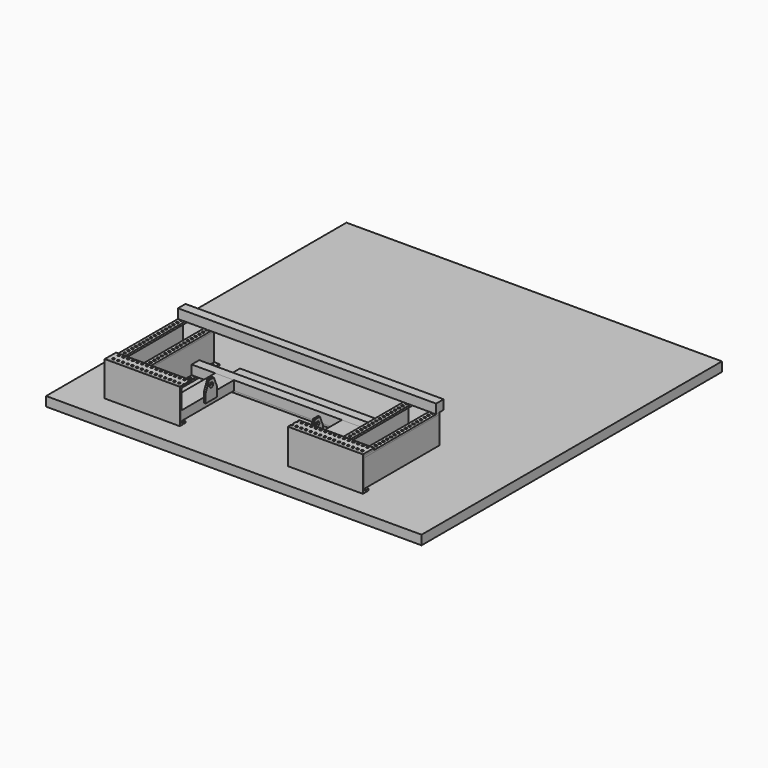
from build123d import *

# Parameters (mm, degrees)
F0_W      = 1016
F0_H      = 1016
F1_DEPTH  = 25.4
F2_W      = 698.5
F2_H      = 88.9
F3_DEPTH  = 5.08
F4_W      = 698.5
F4_H      = 38.1
F4_R      = 3.175
F5_DEPTH  = 5.08
F6_W      = 698.5
F6_H      = 19.05
F6_R      = 3.175
F7_DEPTH  = 5.08
F8_W      = 5.08
F8_H      = 73.66
F9_DEPTH  = 254
F10_W     = 19.05
F10_H     = 254
F10_R     = 3.175
F11_DEPTH = 5.08
F12_W     = 19.05
F12_H     = 254
F12_R     = 3.175
F13_DEPTH = 5.08
F15_W     = 698.5
F15_H     = 25.4
F16_DEPTH = 25.4
F17_W     = 387.35
F17_H     = 254
F18_DEPTH = 12.7
F19_W     = 292.1
F19_H     = 38.1
F20_DEPTH = 165.101
F21_W     = 292.1
F21_H     = 33.02
F22_DEPTH = 63.5
F23_W     = 50.8
F23_H     = 25.4
F24_DEPTH = 177.8
F25_W     = 520.7
F25_H     = 25.4
F26_DEPTH = 25.4
F27_W     = 38.1
F27_H     = 25.4
F27_R     = 6.35
F28_DEPTH = 5.08


with BuildPart() as f1:
    # F0 (on Top) → F1 (new body)
    with BuildSketch(Plane.XY):
        Rectangle(F0_W, F0_H)
    extrude(amount=F1_DEPTH)


with BuildPart() as f3:
    # F2 (on face) → F3 (new body)
    with BuildSketch(Plane.XZ.offset(508)):
        with Locations((0, 120.65)):
            Rectangle(F2_W, F2_H)
    extrude(amount=-F3_DEPTH)

    # F6 (on face) → F7 (join)
    with BuildSketch(Plane(origin=(0, 0, 76.2), x_dir=(1, 0, 0), z_dir=(0, 0, -1))):
        with Locations((0, 498.475)):
            Rectangle(F6_W, F6_H)
        with Locations((-336.55, 495.935)):
            Circle(F6_R, mode=Mode.SUBTRACT)
        with Locations((-323.85, 495.935)):
            Circle(F6_R, mode=Mode.SUBTRACT)
        with Locations((-311.15, 495.935)):
            Circle(F6_R, mode=Mode.SUBTRACT)
        with Locations((-298.45, 495.935)):
            Circle(F6_R, mode=Mode.SUBTRACT)
        with Locations((-285.75, 495.935)):
            Circle(F6_R, mode=Mode.SUBTRACT)
        with Locations((-273.05, 495.935)):
            Circle(F6_R, mode=Mode.SUBTRACT)
        with Locations((-260.35, 495.935)):
            Circle(F6_R, mode=Mode.SUBTRACT)
        with Locations((-247.65, 495.935)):
            Circle(F6_R, mode=Mode.SUBTRACT)
        with Locations((-234.95, 495.935)):
            Circle(F6_R, mode=Mode.SUBTRACT)
        with Locations((-222.25, 495.935)):
            Circle(F6_R, mode=Mode.SUBTRACT)
        with Locations((-209.55, 495.935)):
            Circle(F6_R, mode=Mode.SUBTRACT)
        with Locations((-196.85, 495.935)):
            Circle(F6_R, mode=Mode.SUBTRACT)
        with Locations((-184.15, 495.935)):
            Circle(F6_R, mode=Mode.SUBTRACT)
        with Locations((-171.45, 495.935)):
            Circle(F6_R, mode=Mode.SUBTRACT)
        with Locations((-158.75, 495.935)):
            Circle(F6_R, mode=Mode.SUBTRACT)
        with Locations((-146.05, 495.935)):
            Circle(F6_R, mode=Mode.SUBTRACT)
        with Locations((-133.35, 495.935)):
            Circle(F6_R, mode=Mode.SUBTRACT)
        with Locations((-120.65, 495.935)):
            Circle(F6_R, mode=Mode.SUBTRACT)
        with Locations((-107.95, 495.935)):
            Circle(F6_R, mode=Mode.SUBTRACT)
        with Locations((-95.25, 495.935)):
            Circle(F6_R, mode=Mode.SUBTRACT)
        with Locations((-82.55, 495.935)):
            Circle(F6_R, mode=Mode.SUBTRACT)
        with Locations((-69.85, 495.935)):
            Circle(F6_R, mode=Mode.SUBTRACT)
        with Locations((-57.15, 495.935)):
            Circle(F6_R, mode=Mode.SUBTRACT)
        with Locations((-44.45, 495.935)):
            Circle(F6_R, mode=Mode.SUBTRACT)
        with Locations((-31.75, 495.935)):
            Circle(F6_R, mode=Mode.SUBTRACT)
        with Locations((-19.05, 495.935)):
            Circle(F6_R, mode=Mode.SUBTRACT)
        with Locations((-6.35, 495.935)):
            Circle(F6_R, mode=Mode.SUBTRACT)
        with Locations((6.35, 495.935)):
            Circle(F6_R, mode=Mode.SUBTRACT)
        with Locations((19.05, 495.935)):
            Circle(F6_R, mode=Mode.SUBTRACT)
        with Locations((31.75, 495.935)):
            Circle(F6_R, mode=Mode.SUBTRACT)
        with Locations((44.45, 495.935)):
            Circle(F6_R, mode=Mode.SUBTRACT)
        with Locations((57.15, 495.935)):
            Circle(F6_R, mode=Mode.SUBTRACT)
        with Locations((69.85, 495.935)):
            Circle(F6_R, mode=Mode.SUBTRACT)
        with Locations((82.55, 495.935)):
            Circle(F6_R, mode=Mode.SUBTRACT)
        with Locations((95.25, 495.935)):
            Circle(F6_R, mode=Mode.SUBTRACT)
        with Locations((107.95, 495.935)):
            Circle(F6_R, mode=Mode.SUBTRACT)
        with Locations((120.65, 495.935)):
            Circle(F6_R, mode=Mode.SUBTRACT)
        with Locations((133.35, 495.935)):
            Circle(F6_R, mode=Mode.SUBTRACT)
        with Locations((146.05, 495.935)):
            Circle(F6_R, mode=Mode.SUBTRACT)
        with Locations((158.75, 495.935)):
            Circle(F6_R, mode=Mode.SUBTRACT)
        with Locations((171.45, 495.935)):
            Circle(F6_R, mode=Mode.SUBTRACT)
        with Locations((184.15, 495.935)):
            Circle(F6_R, mode=Mode.SUBTRACT)
        with Locations((196.85, 495.935)):
            Circle(F6_R, mode=Mode.SUBTRACT)
        with Locations((209.55, 495.935)):
            Circle(F6_R, mode=Mode.SUBTRACT)
        with Locations((222.25, 495.935)):
            Circle(F6_R, mode=Mode.SUBTRACT)
        with Locations((234.95, 495.935)):
            Circle(F6_R, mode=Mode.SUBTRACT)
        with Locations((247.65, 495.935)):
            Circle(F6_R, mode=Mode.SUBTRACT)
        with Locations((260.35, 495.935)):
            Circle(F6_R, mode=Mode.SUBTRACT)
        with Locations((273.05, 495.935)):
            Circle(F6_R, mode=Mode.SUBTRACT)
        with Locations((285.75, 495.935)):
            Circle(F6_R, mode=Mode.SUBTRACT)
        with Locations((298.45, 495.935)):
            Circle(F6_R, mode=Mode.SUBTRACT)
        with Locations((311.15, 495.935)):
            Circle(F6_R, mode=Mode.SUBTRACT)
        with Locations((323.85, 495.935)):
            Circle(F6_R, mode=Mode.SUBTRACT)
        with Locations((336.55, 495.935)):
            Circle(F6_R, mode=Mode.SUBTRACT)
    extrude(amount=F7_DEPTH)

    # F8 (on face) → F9 (join)
    with BuildSketch(Plane(origin=(0, -502.92, 0), x_dir=(-1, 0, 0), z_dir=(0, 1, 0))):
        with Locations((-346.71, 118.11)):
            Rectangle(F8_W, F8_H)
        with Locations((-262.89, 118.11)):
            Rectangle(F8_W, F8_H)
    extrude(amount=F9_DEPTH)

    # F12 (on face) → F13 (join)
    with BuildSketch(Plane(origin=(0, 0, 81.28), x_dir=(1, 0, 0), z_dir=(0, 0, -1))):
        with Locations((255.905, 375.92)):
            Rectangle(F12_W, F12_H)
        with Locations((252.73, 261.62)):
            Circle(F12_R, mode=Mode.SUBTRACT)
        with Locations((252.73, 274.32)):
            Circle(F12_R, mode=Mode.SUBTRACT)
        with Locations((252.73, 287.02)):
            Circle(F12_R, mode=Mode.SUBTRACT)
        with Locations((252.73, 299.72)):
            Circle(F12_R, mode=Mode.SUBTRACT)
        with Locations((252.73, 312.42)):
            Circle(F12_R, mode=Mode.SUBTRACT)
        with Locations((252.73, 325.12)):
            Circle(F12_R, mode=Mode.SUBTRACT)
        with Locations((252.73, 337.82)):
            Circle(F12_R, mode=Mode.SUBTRACT)
        with Locations((252.73, 350.52)):
            Circle(F12_R, mode=Mode.SUBTRACT)
        with Locations((252.73, 363.22)):
            Circle(F12_R, mode=Mode.SUBTRACT)
        with Locations((252.73, 375.92)):
            Circle(F12_R, mode=Mode.SUBTRACT)
        with Locations((252.73, 388.62)):
            Circle(F12_R, mode=Mode.SUBTRACT)
        with Locations((252.73, 401.32)):
            Circle(F12_R, mode=Mode.SUBTRACT)
        with Locations((252.73, 414.02)):
            Circle(F12_R, mode=Mode.SUBTRACT)
        with Locations((252.73, 426.72)):
            Circle(F12_R, mode=Mode.SUBTRACT)
        with Locations((252.73, 439.42)):
            Circle(F12_R, mode=Mode.SUBTRACT)
        with Locations((252.73, 452.12)):
            Circle(F12_R, mode=Mode.SUBTRACT)
        with Locations((252.73, 464.82)):
            Circle(F12_R, mode=Mode.SUBTRACT)
        with Locations((252.73, 477.52)):
            Circle(F12_R, mode=Mode.SUBTRACT)
        with Locations((252.73, 490.22)):
            Circle(F12_R, mode=Mode.SUBTRACT)
    extrude(amount=F13_DEPTH)


with BuildPart() as f5:
    # F4 (on face) → F5 (new body)
    with BuildSketch(Plane.XY.offset(165.1)):
        with Locations((0, -488.95)):
            Rectangle(F4_W, F4_H)
        with Locations((-335.4313454818, -495.267126809)):
            Circle(F4_R, mode=Mode.SUBTRACT)
        with Locations((-322.7313454818, -495.267126809)):
            Circle(F4_R, mode=Mode.SUBTRACT)
        with Locations((-310.0313454818, -495.267126809)):
            Circle(F4_R, mode=Mode.SUBTRACT)
        with Locations((-297.3313454818, -495.267126809)):
            Circle(F4_R, mode=Mode.SUBTRACT)
        with Locations((-284.6313454818, -495.267126809)):
            Circle(F4_R, mode=Mode.SUBTRACT)
        with Locations((-271.9313454818, -495.267126809)):
            Circle(F4_R, mode=Mode.SUBTRACT)
        with Locations((-259.2313454818, -495.267126809)):
            Circle(F4_R, mode=Mode.SUBTRACT)
        with Locations((-246.5313454818, -495.267126809)):
            Circle(F4_R, mode=Mode.SUBTRACT)
        with Locations((-233.8313454818, -495.267126809)):
            Circle(F4_R, mode=Mode.SUBTRACT)
        with Locations((-221.1313454818, -495.267126809)):
            Circle(F4_R, mode=Mode.SUBTRACT)
        with Locations((-208.4313454818, -495.267126809)):
            Circle(F4_R, mode=Mode.SUBTRACT)
        with Locations((-195.7313454818, -495.267126809)):
            Circle(F4_R, mode=Mode.SUBTRACT)
        with Locations((-183.0313454818, -495.267126809)):
            Circle(F4_R, mode=Mode.SUBTRACT)
        with Locations((-170.3313454818, -495.267126809)):
            Circle(F4_R, mode=Mode.SUBTRACT)
        with Locations((-157.6313454818, -495.267126809)):
            Circle(F4_R, mode=Mode.SUBTRACT)
        with Locations((-144.9313454818, -495.267126809)):
            Circle(F4_R, mode=Mode.SUBTRACT)
        with Locations((-132.2313454818, -495.267126809)):
            Circle(F4_R, mode=Mode.SUBTRACT)
        with Locations((-119.5313454818, -495.267126809)):
            Circle(F4_R, mode=Mode.SUBTRACT)
        with Locations((-106.8313454818, -495.267126809)):
            Circle(F4_R, mode=Mode.SUBTRACT)
        with Locations((-94.1313454818, -495.267126809)):
            Circle(F4_R, mode=Mode.SUBTRACT)
        with Locations((-81.4313454818, -495.267126809)):
            Circle(F4_R, mode=Mode.SUBTRACT)
        with Locations((-68.7313454818, -495.267126809)):
            Circle(F4_R, mode=Mode.SUBTRACT)
        with Locations((-56.0313454818, -495.267126809)):
            Circle(F4_R, mode=Mode.SUBTRACT)
        with Locations((-43.3313454818, -495.267126809)):
            Circle(F4_R, mode=Mode.SUBTRACT)
        with Locations((-30.6313454818, -495.267126809)):
            Circle(F4_R, mode=Mode.SUBTRACT)
        with Locations((-17.9313454818, -495.267126809)):
            Circle(F4_R, mode=Mode.SUBTRACT)
        with Locations((-5.2313454818, -495.267126809)):
            Circle(F4_R, mode=Mode.SUBTRACT)
        with Locations((7.4686545182, -495.267126809)):
            Circle(F4_R, mode=Mode.SUBTRACT)
        with Locations((20.1686545182, -495.267126809)):
            Circle(F4_R, mode=Mode.SUBTRACT)
        with Locations((32.8686545182, -495.267126809)):
            Circle(F4_R, mode=Mode.SUBTRACT)
        with Locations((45.5686545182, -495.267126809)):
            Circle(F4_R, mode=Mode.SUBTRACT)
        with Locations((58.2686545182, -495.267126809)):
            Circle(F4_R, mode=Mode.SUBTRACT)
        with Locations((70.9686545182, -495.267126809)):
            Circle(F4_R, mode=Mode.SUBTRACT)
        with Locations((83.6686545182, -495.267126809)):
            Circle(F4_R, mode=Mode.SUBTRACT)
        with Locations((96.3686545182, -495.267126809)):
            Circle(F4_R, mode=Mode.SUBTRACT)
        with Locations((109.0686545182, -495.267126809)):
            Circle(F4_R, mode=Mode.SUBTRACT)
        with Locations((121.7686545182, -495.267126809)):
            Circle(F4_R, mode=Mode.SUBTRACT)
        with Locations((134.4686545182, -495.267126809)):
            Circle(F4_R, mode=Mode.SUBTRACT)
        with Locations((147.1686545182, -495.267126809)):
            Circle(F4_R, mode=Mode.SUBTRACT)
        with Locations((159.8686545182, -495.267126809)):
            Circle(F4_R, mode=Mode.SUBTRACT)
        with Locations((172.5686545182, -495.267126809)):
            Circle(F4_R, mode=Mode.SUBTRACT)
        with Locations((185.2686545182, -495.267126809)):
            Circle(F4_R, mode=Mode.SUBTRACT)
        with Locations((197.9686545182, -495.267126809)):
            Circle(F4_R, mode=Mode.SUBTRACT)
        with Locations((210.6686545182, -495.267126809)):
            Circle(F4_R, mode=Mode.SUBTRACT)
        with Locations((223.3686545182, -495.267126809)):
            Circle(F4_R, mode=Mode.SUBTRACT)
        with Locations((236.0686545182, -495.267126809)):
            Circle(F4_R, mode=Mode.SUBTRACT)
        with Locations((248.7686545182, -495.267126809)):
            Circle(F4_R, mode=Mode.SUBTRACT)
        with Locations((261.4686545182, -495.267126809)):
            Circle(F4_R, mode=Mode.SUBTRACT)
        with Locations((274.1686545182, -495.267126809)):
            Circle(F4_R, mode=Mode.SUBTRACT)
        with Locations((286.8686545182, -495.267126809)):
            Circle(F4_R, mode=Mode.SUBTRACT)
        with Locations((299.5686545182, -495.267126809)):
            Circle(F4_R, mode=Mode.SUBTRACT)
        with Locations((312.2686545182, -495.267126809)):
            Circle(F4_R, mode=Mode.SUBTRACT)
        with Locations((324.9686545182, -495.267126809)):
            Circle(F4_R, mode=Mode.SUBTRACT)
        with Locations((337.6686545182, -495.267126809)):
            Circle(F4_R, mode=Mode.SUBTRACT)
        with Locations((-336.55, -476.25)):
            Circle(F4_R, mode=Mode.SUBTRACT)
        with Locations((-323.85, -476.25)):
            Circle(F4_R, mode=Mode.SUBTRACT)
        with Locations((-311.15, -476.25)):
            Circle(F4_R, mode=Mode.SUBTRACT)
        with Locations((-298.45, -476.25)):
            Circle(F4_R, mode=Mode.SUBTRACT)
        with Locations((-285.75, -476.25)):
            Circle(F4_R, mode=Mode.SUBTRACT)
        with Locations((-273.05, -476.25)):
            Circle(F4_R, mode=Mode.SUBTRACT)
        with Locations((-260.35, -476.25)):
            Circle(F4_R, mode=Mode.SUBTRACT)
        with Locations((-247.65, -476.25)):
            Circle(F4_R, mode=Mode.SUBTRACT)
        with Locations((-234.95, -476.25)):
            Circle(F4_R, mode=Mode.SUBTRACT)
        with Locations((-222.25, -476.25)):
            Circle(F4_R, mode=Mode.SUBTRACT)
        with Locations((-209.55, -476.25)):
            Circle(F4_R, mode=Mode.SUBTRACT)
        with Locations((-196.85, -476.25)):
            Circle(F4_R, mode=Mode.SUBTRACT)
        with Locations((-184.15, -476.25)):
            Circle(F4_R, mode=Mode.SUBTRACT)
        with Locations((-171.45, -476.25)):
            Circle(F4_R, mode=Mode.SUBTRACT)
        with Locations((-158.75, -476.25)):
            Circle(F4_R, mode=Mode.SUBTRACT)
        with Locations((-146.05, -476.25)):
            Circle(F4_R, mode=Mode.SUBTRACT)
        with Locations((-133.35, -476.25)):
            Circle(F4_R, mode=Mode.SUBTRACT)
        with Locations((-120.65, -476.25)):
            Circle(F4_R, mode=Mode.SUBTRACT)
        with Locations((-107.95, -476.25)):
            Circle(F4_R, mode=Mode.SUBTRACT)
        with Locations((-95.25, -476.25)):
            Circle(F4_R, mode=Mode.SUBTRACT)
        with Locations((-82.55, -476.25)):
            Circle(F4_R, mode=Mode.SUBTRACT)
        with Locations((-69.85, -476.25)):
            Circle(F4_R, mode=Mode.SUBTRACT)
        with Locations((-57.15, -476.25)):
            Circle(F4_R, mode=Mode.SUBTRACT)
        with Locations((-44.45, -476.25)):
            Circle(F4_R, mode=Mode.SUBTRACT)
        with Locations((-31.75, -476.25)):
            Circle(F4_R, mode=Mode.SUBTRACT)
        with Locations((-19.05, -476.25)):
            Circle(F4_R, mode=Mode.SUBTRACT)
        with Locations((-6.35, -476.25)):
            Circle(F4_R, mode=Mode.SUBTRACT)
        with Locations((6.35, -476.25)):
            Circle(F4_R, mode=Mode.SUBTRACT)
        with Locations((19.05, -476.25)):
            Circle(F4_R, mode=Mode.SUBTRACT)
        with Locations((31.75, -476.25)):
            Circle(F4_R, mode=Mode.SUBTRACT)
        with Locations((44.45, -476.25)):
            Circle(F4_R, mode=Mode.SUBTRACT)
        with Locations((57.15, -476.25)):
            Circle(F4_R, mode=Mode.SUBTRACT)
        with Locations((69.85, -476.25)):
            Circle(F4_R, mode=Mode.SUBTRACT)
        with Locations((82.55, -476.25)):
            Circle(F4_R, mode=Mode.SUBTRACT)
        with Locations((95.25, -476.25)):
            Circle(F4_R, mode=Mode.SUBTRACT)
        with Locations((107.95, -476.25)):
            Circle(F4_R, mode=Mode.SUBTRACT)
        with Locations((120.65, -476.25)):
            Circle(F4_R, mode=Mode.SUBTRACT)
        with Locations((133.35, -476.25)):
            Circle(F4_R, mode=Mode.SUBTRACT)
        with Locations((146.05, -476.25)):
            Circle(F4_R, mode=Mode.SUBTRACT)
        with Locations((158.75, -476.25)):
            Circle(F4_R, mode=Mode.SUBTRACT)
        with Locations((171.45, -476.25)):
            Circle(F4_R, mode=Mode.SUBTRACT)
        with Locations((184.15, -476.25)):
            Circle(F4_R, mode=Mode.SUBTRACT)
        with Locations((196.85, -476.25)):
            Circle(F4_R, mode=Mode.SUBTRACT)
        with Locations((209.55, -476.25)):
            Circle(F4_R, mode=Mode.SUBTRACT)
        with Locations((222.25, -476.25)):
            Circle(F4_R, mode=Mode.SUBTRACT)
        with Locations((234.95, -476.25)):
            Circle(F4_R, mode=Mode.SUBTRACT)
        with Locations((247.65, -476.25)):
            Circle(F4_R, mode=Mode.SUBTRACT)
        with Locations((260.35, -476.25)):
            Circle(F4_R, mode=Mode.SUBTRACT)
        with Locations((273.05, -476.25)):
            Circle(F4_R, mode=Mode.SUBTRACT)
        with Locations((285.75, -476.25)):
            Circle(F4_R, mode=Mode.SUBTRACT)
        with Locations((298.45, -476.25)):
            Circle(F4_R, mode=Mode.SUBTRACT)
        with Locations((311.15, -476.25)):
            Circle(F4_R, mode=Mode.SUBTRACT)
        with Locations((323.85, -476.25)):
            Circle(F4_R, mode=Mode.SUBTRACT)
        with Locations((336.55, -476.25)):
            Circle(F4_R, mode=Mode.SUBTRACT)
    extrude(amount=-F5_DEPTH)


with BuildPart() as f11:
    # F10 (on face) → F11 (new body)
    with BuildSketch(Plane.XY.offset(154.94)):
        with Locations((339.725, -375.92)):
            Rectangle(F10_W, F10_H)
        with Locations((339.725, -490.22)):
            Circle(F10_R, mode=Mode.SUBTRACT)
        with Locations((339.725, -477.52)):
            Circle(F10_R, mode=Mode.SUBTRACT)
        with Locations((339.725, -464.82)):
            Circle(F10_R, mode=Mode.SUBTRACT)
        with Locations((339.725, -452.12)):
            Circle(F10_R, mode=Mode.SUBTRACT)
        with Locations((339.725, -439.42)):
            Circle(F10_R, mode=Mode.SUBTRACT)
        with Locations((339.725, -426.72)):
            Circle(F10_R, mode=Mode.SUBTRACT)
        with Locations((339.725, -414.02)):
            Circle(F10_R, mode=Mode.SUBTRACT)
        with Locations((339.725, -401.32)):
            Circle(F10_R, mode=Mode.SUBTRACT)
        with Locations((339.725, -388.62)):
            Circle(F10_R, mode=Mode.SUBTRACT)
        with Locations((339.725, -375.92)):
            Circle(F10_R, mode=Mode.SUBTRACT)
        with Locations((339.725, -363.22)):
            Circle(F10_R, mode=Mode.SUBTRACT)
        with Locations((339.725, -350.52)):
            Circle(F10_R, mode=Mode.SUBTRACT)
        with Locations((339.725, -337.82)):
            Circle(F10_R, mode=Mode.SUBTRACT)
        with Locations((339.725, -325.12)):
            Circle(F10_R, mode=Mode.SUBTRACT)
        with Locations((339.725, -312.42)):
            Circle(F10_R, mode=Mode.SUBTRACT)
        with Locations((339.725, -299.72)):
            Circle(F10_R, mode=Mode.SUBTRACT)
        with Locations((339.725, -287.02)):
            Circle(F10_R, mode=Mode.SUBTRACT)
        with Locations((339.725, -274.32)):
            Circle(F10_R, mode=Mode.SUBTRACT)
        with Locations((339.725, -261.62)):
            Circle(F10_R, mode=Mode.SUBTRACT)
    extrude(amount=F11_DEPTH)


with BuildPart() as f11b:
    # F10 (on face) → F11, piece 2 (new body)
    with BuildSketch(Plane.XY.offset(154.94)):
        with Locations((269.875, -375.92)):
            Rectangle(F10_W, F10_H)
        with Locations((269.875, -490.22)):
            Circle(F10_R, mode=Mode.SUBTRACT)
        with Locations((269.875, -477.52)):
            Circle(F10_R, mode=Mode.SUBTRACT)
        with Locations((269.875, -464.82)):
            Circle(F10_R, mode=Mode.SUBTRACT)
        with Locations((269.875, -452.12)):
            Circle(F10_R, mode=Mode.SUBTRACT)
        with Locations((269.875, -439.42)):
            Circle(F10_R, mode=Mode.SUBTRACT)
        with Locations((269.875, -426.72)):
            Circle(F10_R, mode=Mode.SUBTRACT)
        with Locations((269.875, -414.02)):
            Circle(F10_R, mode=Mode.SUBTRACT)
        with Locations((269.875, -401.32)):
            Circle(F10_R, mode=Mode.SUBTRACT)
        with Locations((269.875, -388.62)):
            Circle(F10_R, mode=Mode.SUBTRACT)
        with Locations((269.875, -375.92)):
            Circle(F10_R, mode=Mode.SUBTRACT)
        with Locations((269.875, -363.22)):
            Circle(F10_R, mode=Mode.SUBTRACT)
        with Locations((269.875, -350.52)):
            Circle(F10_R, mode=Mode.SUBTRACT)
        with Locations((269.875, -337.82)):
            Circle(F10_R, mode=Mode.SUBTRACT)
        with Locations((269.875, -325.12)):
            Circle(F10_R, mode=Mode.SUBTRACT)
        with Locations((269.875, -312.42)):
            Circle(F10_R, mode=Mode.SUBTRACT)
        with Locations((269.875, -299.72)):
            Circle(F10_R, mode=Mode.SUBTRACT)
        with Locations((269.875, -287.02)):
            Circle(F10_R, mode=Mode.SUBTRACT)
        with Locations((269.875, -274.32)):
            Circle(F10_R, mode=Mode.SUBTRACT)
        with Locations((269.875, -261.62)):
            Circle(F10_R, mode=Mode.SUBTRACT)
    extrude(amount=F11_DEPTH)


with BuildPart() as f14_1:
    # F14: instance of F3
    add(f3.part.mirror(Plane.YZ))


with BuildPart() as f14_2:
    # F14: instance of F11b
    add(f11b.part.mirror(Plane.YZ))


with BuildPart() as f14_3:
    # F14: instance of F11
    add(f11.part.mirror(Plane.YZ))


with BuildPart() as f16:
    # F15 (on face) → F16 (new body)
    with BuildSketch(Plane.XY.offset(160.02)):
        with Locations((0, -247.65)):
            Rectangle(F15_W, F15_H)
    extrude(amount=F16_DEPTH)


with BuildPart() as f18:
    # F17 (on face) → F18 (new body)
    with BuildSketch(Plane.XY.offset(76.2)):
        with Locations((3.175, -375.92)):
            Rectangle(F17_W, F17_H)
    extrude(amount=F18_DEPTH)


with BuildPart() as f20_tool:
    # F19 (on face) → F20 (new body, through all)
    with BuildSketch(Plane.XY.offset(165.1)):
        with Locations((0, -488.95)):
            Rectangle(F19_W, F19_H)
    extrude(amount=-F20_DEPTH)


with BuildPart() as f3_1:
    add(f3.part)

    # F20: cut by f20_tool
    add(f20_tool.part, mode=Mode.SUBTRACT)


with BuildPart() as f5_1:
    add(f5.part)

    # F20: cut by f20_tool
    add(f20_tool.part, mode=Mode.SUBTRACT)


with BuildPart() as f14_1_1:
    add(f14_1.part)

    # F20: cut by f20_tool
    add(f20_tool.part, mode=Mode.SUBTRACT)


with BuildPart() as f18_1:
    add(f18.part)

    # F20: cut by f20_tool
    add(f20_tool.part, mode=Mode.SUBTRACT)

    # F21 (on face) → F22 (cut, through all)
    with BuildSketch(Plane.XY.offset(88.9)):
        with Locations((0, -486.41)):
            Rectangle(F21_W, F21_H)
        Polygon((146.05, -502.92), (196.85, -502.92), (196.85, -325.12), (-190.5, -325.12), (-190.5, -502.92), (-146.05, -502.92), (-146.05, -469.9), (146.05, -469.9), align=None)
    extrude(amount=-F22_DEPTH, mode=Mode.SUBTRACT)


with BuildPart() as f24:
    # F23 (on face) → F24 (new body)
    with BuildSketch(Plane(origin=(0, -502.92, 0), x_dir=(-1, 0, 0), z_dir=(0, 1, 0))):
        with Locations((171.45, 93.98)):
            Rectangle(F23_W, F23_H)
    extrude(amount=F24_DEPTH)

    # F27 (on face) → F28 (join)
    with BuildSketch(Plane.YZ.offset(-146.05)):
        with Locations((-407.67, 106.68)):
            Rectangle(F27_W, F27_H)
        Polygon((-415.8558506179, 144.78), (-426.72, 119.38), (-388.62, 119.38), (-399.4841493821, 144.78), align=None)
        with Locations((-407.67, 130.4520666599)):
            Circle(F27_R, mode=Mode.SUBTRACT)
    extrude(amount=F28_DEPTH)


with BuildPart() as f24b:
    # F23 (on face) → F24, piece 2 (new body)
    with BuildSketch(Plane(origin=(0, -502.92, 0), x_dir=(-1, 0, 0), z_dir=(0, 1, 0))):
        with Locations((-171.45, 93.98)):
            Rectangle(F23_W, F23_H)
    extrude(amount=F24_DEPTH)


with BuildPart() as f26:
    # F25 (on face) → F26 (new body)
    with BuildSketch(Plane(origin=(0, -325.12, 0), x_dir=(-1, 0, 0), z_dir=(0, 1, 0))):
        with Locations((0, 93.98)):
            Rectangle(F25_W, F25_H)
    extrude(amount=F26_DEPTH)


with BuildPart() as f29_1:
    # F29: instance of F24
    add(f24.part.mirror(Plane.YZ))


solid = Compound([f1.part, f11.part, f11b.part, f14_2.part, f14_3.part, f16.part, f3_1.part, f5_1.part, f14_1_1.part, f18_1.part, f24.part, f24b.part, f26.part, f29_1.part])
